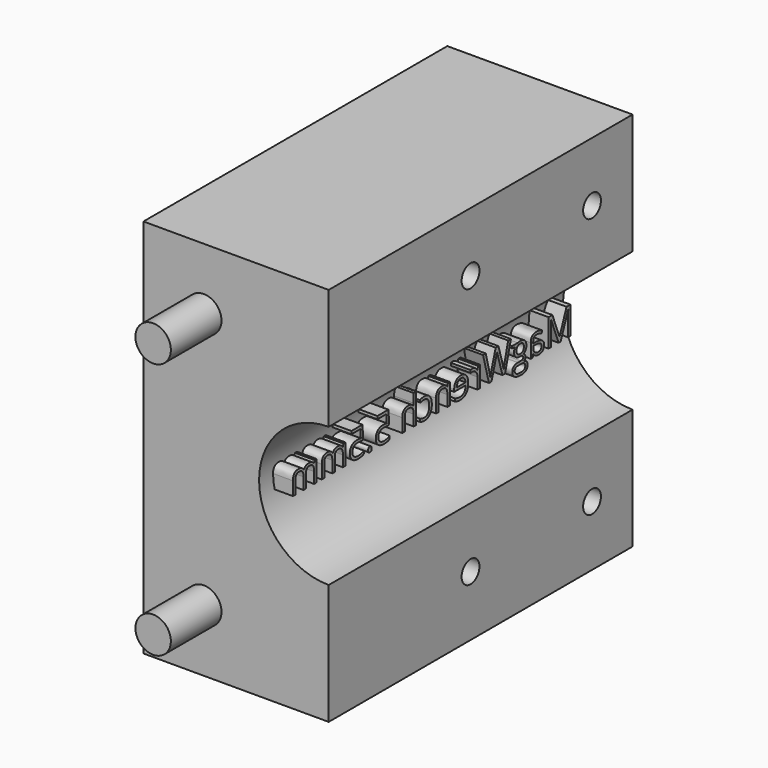
from build123d import *

# Parameters (mm, degrees)
F1_DEPTH      = 38.1
F2_R          = 1.1176
F3_DEPTH      = 6.35
F5_R          = 1.778
F6_DEPTH      = 6.35
F7_R          = 1.905
F8_DEPTH      = 6.35
F13_TEXT_SIZE = 3.8852882692
F14_DEPTH     = 2


# Not quite as in the source:
# - Text() gives the source's letters only with a copy of the font that has no kerning and outlines rounded to 1/6400 em; it was checked with that copy


with BuildPart() as f1:
    # F0 (on Front) → F1 (new body)
    with BuildSketch(Plane.XZ):
        with BuildLine():
            ThreePointArc((0, -6.985), (-6.985, 0), (0, 6.985))
            Line((0, 6.985), (0, 19.0754))
            Line((0, 19.0754), (-18.5835938901, 19.0754))
            Line((-18.5835938901, 19.0754), (-18.5835938901, -19.0754))
            Line((-18.5835938901, -19.0754), (0, -19.0754))
            Line((0, -19.0754), (0, -6.985))
        make_face()
    extrude(amount=F1_DEPTH)

    # F2 (on Right) → F3 (cut)
    with BuildSketch(Plane.YZ):
        with Locations((-20.3159409893, 13.0939871032)):
            Circle(F2_R)
        with Locations((-5.08, 13.0939871032)):
            Circle(F2_R)
        with Locations((-20.3159409893, -13.0351273384)):
            Circle(F2_R)
        with Locations((-5.08, -13.0351273384)):
            Circle(F2_R)
    extrude(amount=-F3_DEPTH, mode=Mode.SUBTRACT)


with BuildPart() as f4_1:
    # F4: copy of F1
    add(f1.part)


with BuildPart() as f6:
    # F5 (on face) → F6 (new body)
    with BuildSketch(Plane.XZ.offset(38.1)):
        with Locations((-12.5311835162, 12.8628154198)):
            Circle(F5_R)
    extrude(amount=F6_DEPTH)


with BuildPart() as f6b:
    # F5 (on face) → F6, piece 2 (new body)
    with BuildSketch(Plane.XZ.offset(38.1)):
        with Locations((-12.5311835162, -12.8628154198)):
            Circle(F5_R)
    extrude(amount=F6_DEPTH)


with BuildPart() as f8:
    # F7 (on face) → F8 (new body)
    with BuildSketch(Plane(origin=(0, 0, 0), x_dir=(-1, 0, 0), z_dir=(0, 1, 0))):
        with Locations((12.5311835162, 12.8628154198)):
            Circle(F7_R)
    extrude(amount=F8_DEPTH)


with BuildPart() as f8b:
    # F7 (on face) → F8, piece 2 (new body)
    with BuildSketch(Plane(origin=(0, 0, 0), x_dir=(-1, 0, 0), z_dir=(0, 1, 0))):
        with Locations((12.5311835162, -12.8628154198)):
            Circle(F7_R)
    extrude(amount=F8_DEPTH)


with BuildPart() as f14:
    # F13 (on face) → F14 (new body)
    with BuildSketch(Plane(origin=(-6.985, 0, 0), x_dir=(0, -1, 0), z_dir=(-1, 0, 0))):
        with Locations((1.1754508596, -1.4685176939)):
            Text('MagWrench 5.5mm', F13_TEXT_SIZE, font='Open Sans', text_align=(TextAlign.LEFT, TextAlign.BOTTOM))
    extrude(amount=-F14_DEPTH)


solid = Compound([f1.part, f4_1.part, f6.part, f6b.part, f8.part, f8b.part, f14.part])
